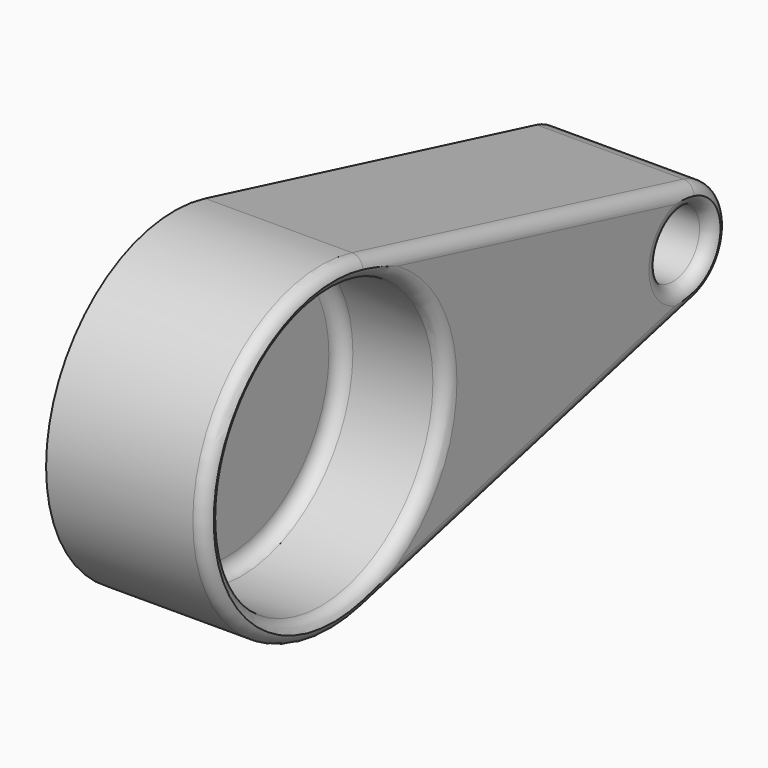
from build123d import *

# Parameters (mm, degrees)
F1_DEPTH = 76.2
F2_R     = 66.675
F2_R_2   = 15.875
F3_DEPTH = 50.8
F4_F1_R  = 6.35
F4_F2_R  = 6.35
F4_F3_R  = 6.35
F5_T     = -2.54


# Not quite as in the source:
# - a fillet or chamfer that OpenCascade refuses, or shapes differently, is made with other operations: its cross-section is extruded or revolved along the edge and cut away or added


with BuildPart() as f1:
    # F0 (on Right) → F1 (new body)
    with BuildSketch(Plane.YZ):
        with BuildLine():
            ThreePointArc((18.4812146278, 73.9248585111), (60.0612543768, 46.8944103565), (76.2, 0))
            ThreePointArc((76.2, 0), (60.0612543768, -46.8944103565), (18.4812146278, -73.9248585111))
            Line((18.4812146278, -73.9248585111), (215.6141706573, -24.6416195037))
            ThreePointArc((215.6141706573, -24.6416195037), (184.0537657814, 0), (215.6141706573, 24.6416195037))
            Line((215.6141706573, 24.6416195037), (18.4812146278, 73.9248585111))
        make_face()
        with BuildLine():
            ThreePointArc((18.4812146278, -73.9248585111), (60.0612543768, -46.8944103565), (76.2, 0))
            ThreePointArc((76.2, 0), (60.0612543768, 46.8944103565), (18.4812146278, 73.9248585111))
            ThreePointArc((18.4812146278, 73.9248585111), (-76.2, 0), (18.4812146278, -73.9248585111))
        make_face()
        with BuildLine():
            ThreePointArc((234.8537657814, 0), (229.474183907, 15.6314701188), (215.6141706573, 24.6416195037))
            ThreePointArc((215.6141706573, 24.6416195037), (184.0537657814, 0), (215.6141706573, -24.6416195037))
            ThreePointArc((215.6141706573, -24.6416195037), (229.474183907, -15.6314701188), (234.8537657814, 0))
        make_face()
    extrude(amount=F1_DEPTH)

    # F2 (on face) → F3 (cut)
    with BuildSketch(Plane.YZ.offset(76.2)):
        Circle(F2_R)
        with Locations((209.4537657814, 0)):
            Circle(F2_R_2)
    extrude(amount=-F3_DEPTH, mode=Mode.SUBTRACT)

    # F4: fillet of radius 6.35 on 10 edges, made by hand

    # F4_f1
    f4_f1_edges = [f1.edges().sort_by_distance(p)[0] for p in [
        (76.2, 117.0476926425, 49.2832390074),
        (76.2, 234.8537657814, 0),
        (76.2, -76.2, 0),
        (76.2, 117.0476926425, -49.2832390074),
    ]]
    fillet(f4_f1_edges, radius=F4_F1_R)

    # F4_f2
    f4_f2_edges = [f1.edges().sort_by_distance(p)[0] for p in [
        (25.4, -66.675, 0),
    ]]
    fillet(f4_f2_edges, radius=F4_F2_R)

    # F4_f3
    f4_f3_edges = [f1.edges().sort_by_distance(p)[0] for p in [
        (25.4, 193.5787657814, 0),
    ]]
    fillet(f4_f3_edges, radius=F4_F3_R)

    # F4_s4 → F4_t5 (revolve, cut)
    with BuildSketch(Plane.XY):
        with BuildLine():
            ThreePointArc((76.2, 73.025), (74.3401280605, 68.5348719395), (69.85, 66.675))
            Line((69.85, 66.675), (69.85, 66.548))
            Line((69.85, 66.548), (76.327, 66.548))
            Line((76.327, 66.548), (76.327, 73.025))
            Line((76.327, 73.025), (76.2, 73.025))
        make_face()
    revolve(axis=Axis((76.2, 0, 0), (1, 0, 0)), mode=Mode.SUBTRACT)

    # F4_s6 → F4_t7 (revolve, cut)
    with BuildSketch(Plane.XY):
        with BuildLine():
            ThreePointArc((69.85, 225.3287657814), (74.3401280605, 227.1886377208), (76.2, 231.6787657814))
            Line((76.2, 231.6787657814), (76.327, 231.6787657814))
            Line((76.327, 231.6787657814), (76.327, 225.2017657814))
            Line((76.327, 225.2017657814), (69.85, 225.2017657814))
            Line((69.85, 225.2017657814), (69.85, 225.3287657814))
        make_face()
    revolve(axis=Axis((76.2, 209.4537657814, 0), (1, 0, 0)), mode=Mode.SUBTRACT)

    # F5
    f5_openings = [f1.faces().sort_by_distance(p)[0] for p in [
        (0, 57.51924, 0),
    ]]
    offset(amount=F5_T, openings=f5_openings)


solid = f1.part
